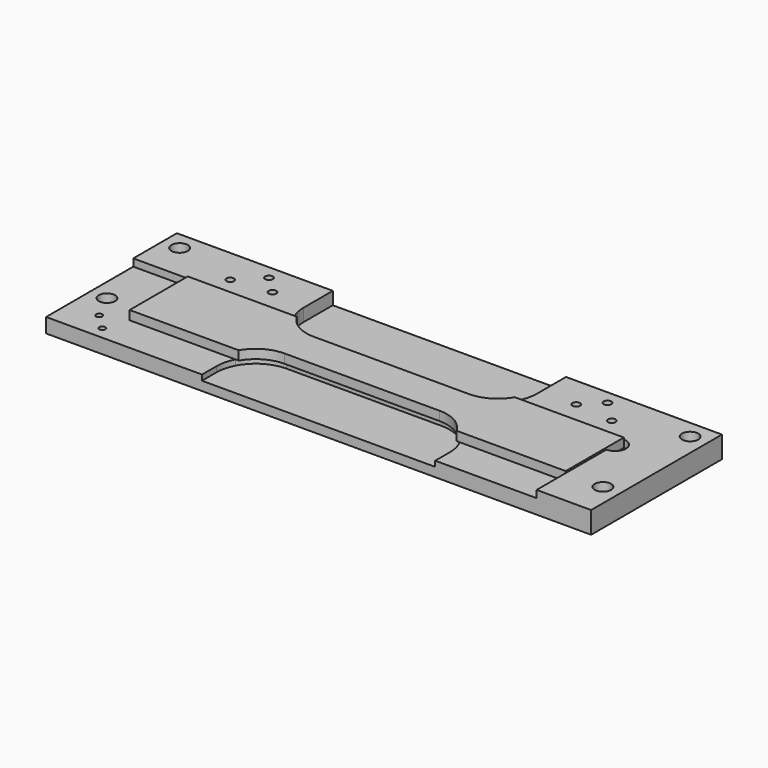
from build123d import *

# Parameters (mm, degrees)
F1_DEPTH  = 5
F3_DEPTH  = 3
F4_W      = 20
F4_H      = 60
F5_DEPTH  = 5
F6_DEPTH  = 4
F7_DEPTH  = 20
F8_R      = 2.1
F9_DEPTH  = 25
F10_R     = 4.5
F11_DEPTH = 25
F13_DEPTH = 10
F12_R     = 1.7
F14_DEPTH = 25


# Not quite as in the source:
# - a feature names something its author has since deleted; it is built from what else it names


with BuildPart() as f1:
    # F0 (on Top) → F1 (new body)
    with BuildSketch(Plane.XY):
        with BuildLine():
            Line((0, -10), (0, 0))
            Line((0, 0), (120, 0))
            Line((120, 0), (120, 20))
            Line((120, 20), (60, 20))
            ThreePointArc((60, 20), (52.6794919243, 12.6794919243), (42.6794919243, 10))
            Line((42.6794919243, 10), (0, 10))
            Line((0, 10), (-42.6794919243, 10))
            ThreePointArc((-42.6794919243, 10), (-52.6794919243, 12.6794919243), (-60, 20))
            Line((-60, 20), (-120, 20))
            Line((-120, 20), (-120, 0))
            Line((-120, 0), (-120, -20))
            Line((-120, -20), (-60, -20))
            ThreePointArc((-60, -20), (-52.6794919243, -12.6794919243), (-42.6794919243, -10))
            Line((-42.6794919243, -10), (0, -10))
        make_face()
        with BuildLine():
            Line((120, 0), (0, 0))
            Line((0, 0), (0, -10))
            Line((0, -10), (42.6794919243, -10))
            ThreePointArc((42.6794919243, -10), (52.6794919243, -12.6794919243), (60, -20))
            Line((60, -20), (120, -20))
            Line((120, -20), (120, 0))
        make_face()
    extrude(amount=F1_DEPTH)


with BuildPart() as f3:
    # F2 (on face) → F3 (new body)
    with BuildSketch(Plane(origin=(0, 0, 0), x_dir=(1, 0, 0), z_dir=(0, 0, -1))):
        with BuildLine():
            Line((120, 30), (64.1794919243, 30))
            ThreePointArc((64.1794919243, 30), (63.5535982007, 24.8500789171), (61.712358235, 20))
            Line((61.712358235, 20), (120, 20))
            Line((120, 20), (120, 30))
        make_face()
        with BuildLine():
            Line((120, 20), (61.712358235, 20))
            ThreePointArc((61.712358235, 20), (53.7981699033, 11.5982337804), (42.6794919243, 8.5))
            Line((42.6794919243, 8.5), (-42.6794919243, 8.5))
            ThreePointArc((-42.6794919243, 8.5), (-53.7981699033, 11.5982337804), (-61.712358235, 20))
            Line((-61.712358235, 20), (-120, 20))
            Line((-120, 20), (-120, -20))
            Line((-120, -20), (-61.712358235, -20))
            ThreePointArc((-61.712358235, -20), (-53.7981699033, -11.5982337804), (-42.6794919243, -8.5))
            Line((-42.6794919243, -8.5), (42.6794919243, -8.5))
            ThreePointArc((42.6794919243, -8.5), (53.7981699033, -11.5982337804), (61.712358235, -20))
            Line((61.712358235, -20), (120, -20))
            Line((120, -20), (120, -8))
            Line((120, -8), (120, 20))
        make_face()
        with BuildLine():
            ThreePointArc((-61.712358235, 20), (-63.5535982007, 24.8500789171), (-64.1794919243, 30))
            Line((-64.1794919243, 30), (-150, 30))
            Line((-150, 30), (-150, -20))
            Line((-150, -20), (-120, -20))
            Line((-120, -20), (-120, 20))
            Line((-120, 20), (-61.712358235, 20))
        make_face()
        with BuildLine():
            Line((-120, -20), (-150, -20))
            Line((-150, -20), (-150, -30))
            Line((-150, -30), (-64.1794919243, -30))
            ThreePointArc((-64.1794919243, -30), (-63.5535982007, -24.8500789171), (-61.712358235, -20))
            Line((-61.712358235, -20), (-120, -20))
        make_face()
        with BuildLine():
            Line((150, 30), (120, 30))
            Line((120, 30), (120, 20))
            Line((120, 20), (120, -8))
            ThreePointArc((120, -8), (126, -14), (120, -20))
            Line((120, -20), (61.712358235, -20))
            ThreePointArc((61.712358235, -20), (63.5535982007, -24.8500789171), (64.1794919243, -30))
            Line((64.1794919243, -30), (150, -30))
            Line((150, -30), (150, 30))
        make_face()
        with BuildLine():
            ThreePointArc((120, -20), (126, -14), (120, -8))
            Line((120, -8), (120, -20))
        make_face()
    extrude(amount=F3_DEPTH)

    # F4 (on face) → F5 (join)
    with BuildSketch(Plane(origin=(0, 0, -3), x_dir=(1, 0, 0), z_dir=(0, 0, -1))):
        with BuildLine():
            Line((64.1794919243, -30), (130, -30))
            Line((130, -30), (130, 30))
            Line((130, 30), (64.1794919243, 30))
            ThreePointArc((64.1794919243, 30), (57.8822877198, 14.7972042045), (42.6794919243, 8.5))
            Line((42.6794919243, 8.5), (-42.6794919243, 8.5))
            ThreePointArc((-42.6794919243, 8.5), (-57.8822877198, 14.7972042045), (-64.1794919243, 30))
            Line((-64.1794919243, 30), (-130, 30))
            Line((-130, 30), (-130, -30))
            Line((-130, -30), (-64.1794919243, -30))
            ThreePointArc((-64.1794919243, -30), (-57.8822877198, -14.7972042045), (-42.6794919243, -8.5))
            Line((-42.6794919243, -8.5), (42.6794919243, -8.5))
            ThreePointArc((42.6794919243, -8.5), (57.8822877198, -14.7972042045), (64.1794919243, -30))
        make_face()
        with BuildLine():
            ThreePointArc((42.6794919243, 8.5), (57.8822877198, 14.7972042045), (64.1794919243, 30))
            Line((64.1794919243, 30), (-64.1794919243, 30))
            ThreePointArc((-64.1794919243, 30), (-57.8822877198, 14.7972042045), (-42.6794919243, 8.5))
            Line((-42.6794919243, 8.5), (42.6794919243, 8.5))
        make_face()
        with BuildLine():
            Line((-64.1794919243, -30), (64.1794919243, -30))
            ThreePointArc((64.1794919243, -30), (57.8822877198, -14.7972042045), (42.6794919243, -8.5))
            Line((42.6794919243, -8.5), (-42.6794919243, -8.5))
            ThreePointArc((-42.6794919243, -8.5), (-57.8822877198, -14.7972042045), (-64.1794919243, -30))
        make_face()
        with Locations((-140, 0)):
            Rectangle(F4_W, F4_H)
        with Locations((140, 0)):
            Rectangle(F4_W, F4_H)
    extrude(amount=F5_DEPTH)

    # F2 (on face) → F6 (join)
    with BuildSketch(Plane(origin=(0, 0, 0), x_dir=(1, 0, 0), z_dir=(0, 0, -1))):
        with BuildLine():
            Line((150, 30), (120, 30))
            Line((120, 30), (120, 20))
            Line((120, 20), (120, -8))
            ThreePointArc((120, -8), (126, -14), (120, -20))
            Line((120, -20), (61.712358235, -20))
            ThreePointArc((61.712358235, -20), (63.5535982007, -24.8500789171), (64.1794919243, -30))
            Line((64.1794919243, -30), (150, -30))
            Line((150, -30), (150, 30))
        make_face()
        with BuildLine():
            Line((-120, -20), (-150, -20))
            Line((-150, -20), (-150, -30))
            Line((-150, -30), (-64.1794919243, -30))
            ThreePointArc((-64.1794919243, -30), (-63.5535982007, -24.8500789171), (-61.712358235, -20))
            Line((-61.712358235, -20), (-120, -20))
        make_face()
    extrude(amount=-F6_DEPTH)

    # F7 (add): a face of the model
    f7_faces = [f3.faces().sort_by_distance(p)[0] for p in [
        (67.1818909651, 30, 0.5),
    ]]
    extrude(f7_faces, amount=F7_DEPTH)

    # F8 (on face) → F9 (cut)
    with BuildSketch(Plane.XY.offset(4)):
        with Locations((-105.0294919243, 30.44)):
            Circle(F8_R)
        with Locations((-93.1494919243, 42.32)):
            Circle(F8_R)
        with Locations((-83.5994919243, 32.78)):
            Circle(F8_R)
        with Locations((83.5994919243, 32.78)):
            Circle(F8_R)
        with Locations((93.1494919243, 42.32)):
            Circle(F8_R)
        with Locations((105.0294919243, 30.44)):
            Circle(F8_R)
    extrude(amount=-F9_DEPTH, mode=Mode.SUBTRACT)

    # F10 (on face) → F11 (cut)
    with BuildSketch(Plane.XY.offset(5)):
        with Locations((-140.5, -10)):
            Circle(F10_R)
        with Locations((140.5, -20)):
            Circle(F10_R)
        with Locations((-140.5, 40)):
            Circle(F10_R)
        with Locations((140.5, 40)):
            Circle(F10_R)
    extrude(amount=-F11_DEPTH, mode=Mode.SUBTRACT)

    # F13 (add): a face of the model
    f13_faces = [f3.faces().sort_by_distance(p)[0] for p in [
        (7.5880955109, -30, -4.1136773426),
    ]]
    extrude(f13_faces, amount=F13_DEPTH)

    # F12 (on face) → F14 (cut)
    with BuildSketch(Plane.XY):
        with Locations((-124.59, -33.07)):
            Circle(F12_R)
        with Locations((-133.07, -24.59)):
            Circle(F12_R)
    extrude(amount=-F14_DEPTH, mode=Mode.SUBTRACT)


solid = Compound([f1.part, f3.part])
